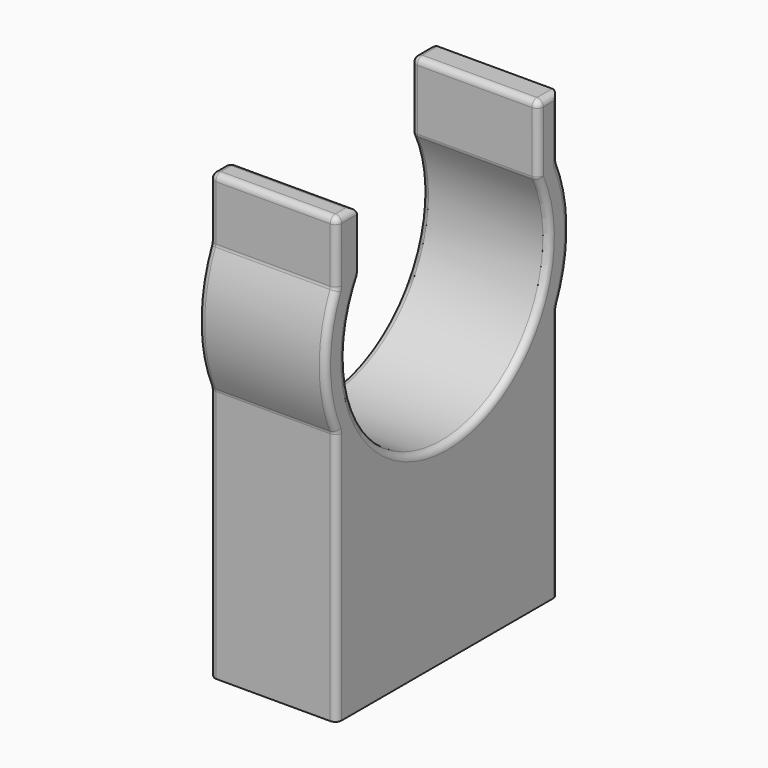
from build123d import *

# Parameters (mm, degrees)
F1_DEPTH = 12.7
F2_F1_R  = 1.27
F2_F2_R  = 1.27


with BuildPart() as f1:
    # F0 (on Right) → F1 (new body, symmetric)
    with BuildSketch(Plane.YZ):
        with BuildLine():
            ThreePointArc((-22.86, -11.0716033166), (-25.3986752482, 0.259414025), (-22.6290909091, 11.5362144843))
            Line((-22.6290909091, 11.5362144843), (-22.6290909091, 25.197786356))
            Line((-22.6290909091, 25.197786356), (-27.7090909091, 25.197786356))
            Line((-27.7090909091, 25.197786356), (-27.7090909091, 12.6979006529))
            ThreePointArc((-27.7090909091, 12.6979006529), (-30.48, 0), (-27.7090909091, -12.6979006529))
            Line((-27.7090909091, -12.6979006529), (-27.7090909091, -63.5))
            Line((-27.7090909091, -63.5), (-22.86, -63.5))
            Line((-22.86, -63.5), (22.86, -63.5))
            Line((22.86, -63.5), (27.7090909091, -63.5))
            Line((27.7090909091, -63.5), (27.7090909091, -12.6979006529))
            ThreePointArc((27.7090909091, -12.6979006529), (30.48, 0), (27.7090909091, 12.6979006529))
            Line((27.7090909091, 12.6979006529), (27.7090909091, 25.197786356))
            Line((27.7090909091, 25.197786356), (22.6290909091, 25.197786356))
            Line((22.6290909091, 25.197786356), (22.6290909091, 11.5362144843))
            ThreePointArc((22.6290909091, 11.5362144843), (25.3986752482, 0.259414025), (22.86, -11.0716033166))
            ThreePointArc((22.86, -11.0716033166), (0, -25.4), (-22.86, -11.0716033166))
        make_face()
    extrude(amount=F1_DEPTH, both=True)

    # F2: fillet of radius 1.27 on 31 edges, made by hand

    # F2_f1
    f2_f1_edges = [f1.edges().sort_by_distance(p)[0] for p in [
        (0, 27.7090909091, 12.6979006529),
        (0, 27.7090909091, -12.6979006529),
        (0, -27.7090909091, 12.6979006529),
        (0, -27.7090909091, -12.6979006529),
    ]]
    fillet(f2_f1_edges, radius=F2_F1_R)

    # F2_f2
    f2_f2_edges = [f1.edges().sort_by_distance(p)[0] for p in [
        (0, -22.6290909091, 25.197786356),
        (0, -27.7090909091, 25.197786356),
        (-12.7, -25.1690909091, 25.197786356),
        (12.7, -25.1690909091, 25.197786356),
        (12.7, 25.1690909091, 25.197786356),
        (-12.7, 25.1690909091, 25.197786356),
        (0, 22.6290909091, 25.197786356),
        (-6.35, -22.6290909091, 11.5362144843),
        (6.35, -22.6290909091, 11.5362144843),
        (-6.35, 22.6290909091, 11.5362144843),
        (6.35, 22.6290909091, 11.5362144843),
        (-12.7, -27.7090909091, -38.2360386617),
        (-12.7, 27.7090909091, 19.0849318397),
        (-12.7, 22.6290909091, 18.3670004202),
        (-12.7, 25.3986752482, 0.259414025),
        (-12.7, 0, -25.4),
        (-12.7, -25.3986752482, 0.259414025),
        (-12.7, -22.6290909091, 18.3670004202),
        (-12.7, -27.7090909091, 19.0849318397),
        (-12.7, -30.48, 0),
        (-12.7, 0, -63.5),
        (-12.7, 27.7090909091, -38.2360386617),
        (-12.7, 30.48, 0),
        (12.7, -30.48, 0),
        (12.7, 0, -25.4),
        (12.7, 30.48, 0),
        (12.7, 22.6290909091, 18.3670004202),
        (12.7, 25.3986752482, 0.259414025),
        (12.7, -25.3986752482, 0.259414025),
        (12.7, 27.7371090618, -12.7067829757),
        (12.7, 27.7371090618, 12.7067829757),
        (12.7, -27.7371090618, 12.7067829757),
        (12.7, -27.7371090618, -12.7067829757),
        (-12.7, 27.7371090618, -12.7067829757),
        (-12.7, 27.7371090618, 12.7067829757),
        (-12.7, -27.7371090618, 12.7067829757),
        (-12.7, -27.7371090618, -12.7067829757),
    ]]
    fillet(f2_f2_edges, radius=F2_F2_R)


solid = f1.part
